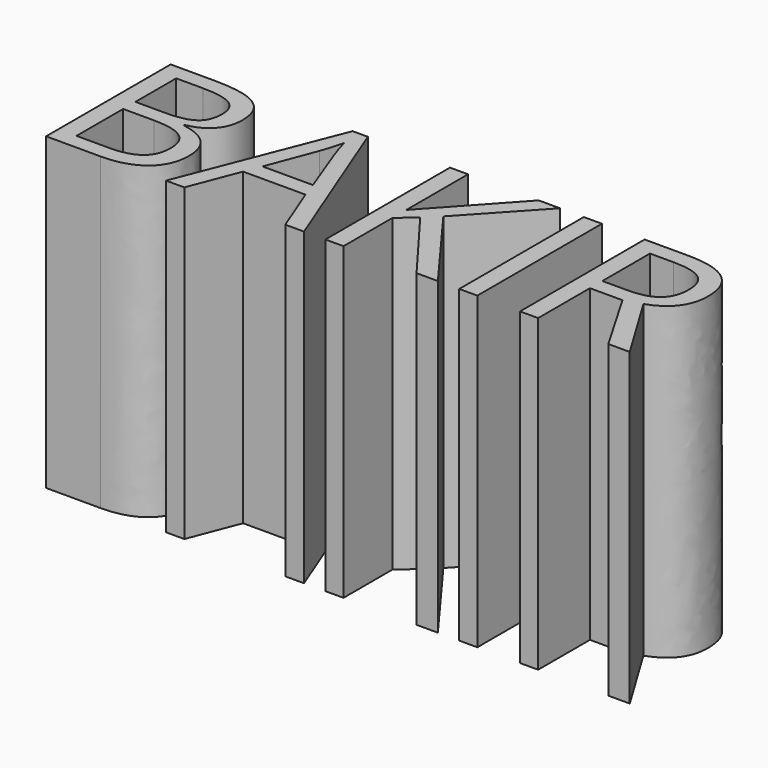
from build123d import *

# Parameters (mm, degrees)
F0_TEXT_SIZE = 35.2209564691
F1_DEPTH     = 50


# Not quite as in the source:
# - Text() gives the source's letters only with a copy of the font that has no kerning and outlines rounded to 1/6400 em; it was checked with that copy


with BuildPart() as f1:
    # F0 (on Top) → F1 (new body)
    with BuildSketch(Plane.XY):
        with Locations((-68.6444190385, 27.5452122903)):
            Text('BAKIR', F0_TEXT_SIZE, font='Open Sans', text_align=(TextAlign.LEFT, TextAlign.BOTTOM))
    extrude(amount=-F1_DEPTH)


solid = f1.part
